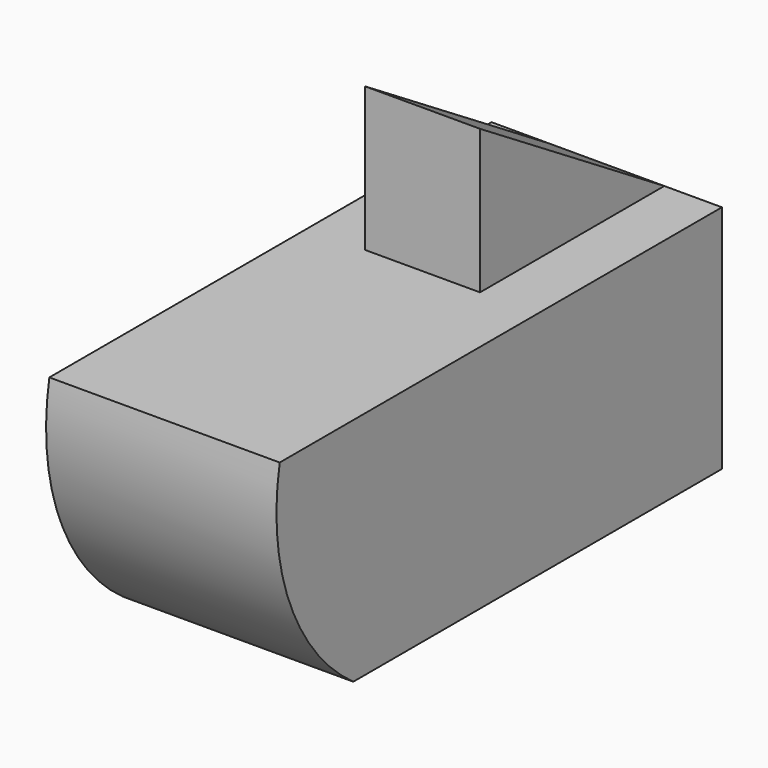
from build123d import *

# Parameters (mm, degrees)
F1_DEPTH = 20
F3_DEPTH = 10


# Not quite as in the source:
# - a feature of the source that left no trace in its solid (it failed there, or was rolled back) is left out


with BuildPart() as f1:
    # F0 (on Right) → F1 (new body, symmetric)
    with BuildSketch(Plane.YZ):
        Polygon((-27.5, 18.3739837377), (-40, 18.3739837377), (-40, -21.6260162623), (40, -21.6260162623), (40, 18.3739837377), (11.153018102, 18.3739837377), (0, 18.3739837377), (-5, 18.3739837377), (-17.5, 18.3739837377), align=None)
        with BuildLine():
            Line((-40, -21.6260162623), (-40, 18.3739837377))
            Line((-40, 18.3739837377), (-50.9159490466, 18.3739837377))
            Line((-50.9159490466, 18.3739837377), (-55.972136481, 18.3739837377))
            ThreePointArc((-55.972136481, 18.3739837377), (-53.829536351, -3.9593330169), (-40, -21.6260162623))
        make_face()
    extrude(amount=F1_DEPTH, both=True)

    # F0 (on Right) → F3 (join, symmetric)
    with BuildSketch(Plane.YZ):
        Polygon((11.153018102, 18.3739837377), (40, 18.3739837377), (0, 43.3739837377), (0, 18.3739837377), align=None)
    extrude(amount=F3_DEPTH, both=True)


solid = f1.part
